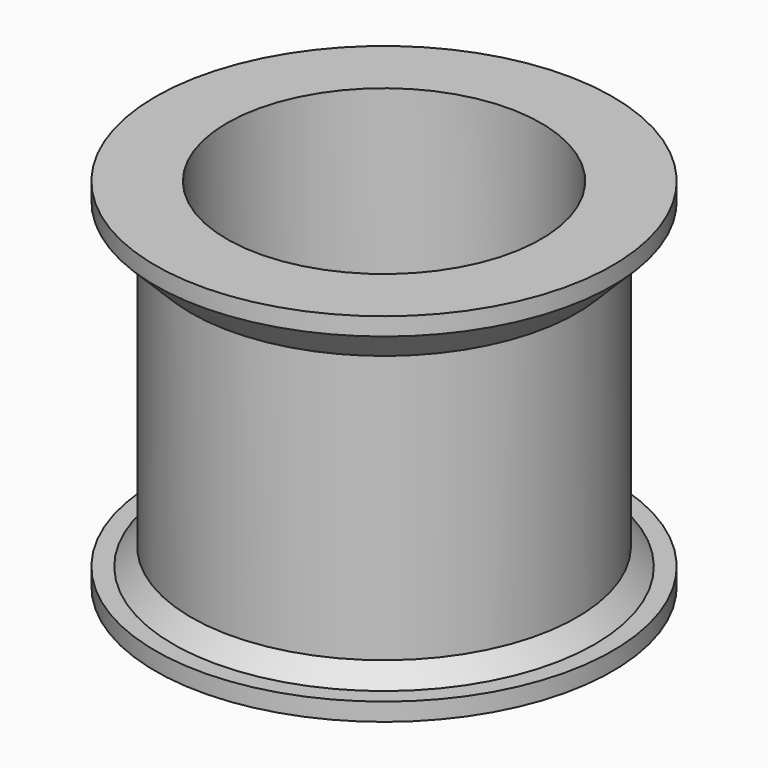
from build123d import *

# Parameters (mm, degrees)
F0_R     = 15.875
F0_R_2   = 4.318
F1_DEPTH = 11.43
F5_SIZE  = 1.5875
F4_R     = 15.875
F4_R_2   = 13.97
F6_DEPTH = 3.175


with BuildPart() as f1:
    # F0 (on Top) → F1 (new body)
    with BuildSketch(Plane.XY):
        Circle(F0_R)
        Circle(F0_R_2, mode=Mode.SUBTRACT)
    extrude(amount=F1_DEPTH)

    # F2 (on Front) → F3 (revolve)
    with BuildSketch(Plane.XZ):
        Polygon((-20.32, 0), (-10.16, 0), (-10.16, 1.5875), (-13.97, 1.5875), (-13.97, 31.75), (-20.32, 31.75), (-20.32, 30.1625), (-17.145, 30.1625), (-17.145, 26.9875), (-17.145, 1.5875), (-20.32, 1.5875), align=None)
        Polygon((-20.32, 30.1625), (-17.145, 26.9875), (-17.145, 30.1625), align=None)
    revolve(axis=Axis((0, 0, 11.5776285529), (0, 0, 1)))

    # F5
    f5_edges = [f1.edges().sort_by_distance(p)[0] for p in [
        (17.145, 0, 1.5875),
    ]]
    chamfer(f5_edges, length=F5_SIZE)

    # F4 (on face) → F6 (join)
    with BuildSketch(Plane.XY.offset(11.43)):
        Circle(F4_R)
        Circle(F4_R_2, mode=Mode.SUBTRACT)
        Circle(F4_R_2)
        with BuildLine():
            ThreePointArc((0, 13.49375), (1.9203608066, 13.3564030875), (3.8016286067, 12.9471583368))
            ThreePointArc((3.8016286067, 12.9471583368), (7.2952719665, 11.3516648998), (10.1978957754, 8.836527079))
            ThreePointArc((10.1978957754, 8.836527079), (12.2743466965, 5.6055064211), (13.3564030629, 1.9203609777))
            ThreePointArc((13.3564030629, 1.9203609777), (13.4593694669, 0.9626331682), (13.49375, 0))
            ThreePointArc((13.49375, 0), (13.1853755264, -2.8683028589), (12.2743467518, -5.6055063))
            ThreePointArc((12.2743467518, -5.6055063), (10.197895881, -8.836526957), (7.2952721608, -11.3516647749))
            ThreePointArc((7.2952721608, -11.3516647749), (3.8016288023, -12.9471582794), (8.16e-08, -13.49375))
            ThreePointArc((8.16e-08, -13.49375), (-3.8016286419, -12.9471583265), (-7.2952720168, -11.3516648675))
            ThreePointArc((-7.2952720168, -11.3516648675), (-10.1978957807, -8.8365270728), (-12.2743466957, -5.6055064229))
            ThreePointArc((-12.2743466957, -5.6055064229), (-13.3564030713, -1.920360919), (-13.3564030873, 1.9203608081))
            ThreePointArc((-13.3564030873, 1.9203608081), (-12.2743467595, 5.6055062831), (-10.1978958619, 8.8365269791))
            ThreePointArc((-10.1978958619, 8.8365269791), (-7.2952721155, 11.3516648041), (-3.8016288198, 12.9471582743))
            ThreePointArc((-3.8016288198, 12.9471582743), (-1.9203609165, 13.3564030717), (0, 13.49375))
        make_face(mode=Mode.SUBTRACT)
        with BuildLine():
            ThreePointArc((10.1978957754, 8.836527079), (7.2952719665, 11.3516648998), (3.8016286067, 12.9471583368))
            ThreePointArc((3.8016286067, 12.9471583368), (4.0909657389, 12.766807831), (4.2453187505, 12.462805481))
            Line((4.2453187505, 12.462805481), (4.8828478786, 9.2855481142))
            ThreePointArc((4.8828478786, 9.2855481142), (6.002488465, 10.799178406), (7.3980285057, 9.5353984813))
            ThreePointArc((7.3980285057, 9.5353984813), (7.1233157795, 8.7465364892), (6.4180233992, 8.2989507623))
            Line((6.4180233992, 8.2989507623), (9.572997339, 9.0389143838))
            ThreePointArc((9.572997339, 9.0389143838), (9.9136481809, 9.0247970952), (10.1978957754, 8.836527079))
        make_face()
        with BuildLine():
            ThreePointArc((13.3564030629, 1.9203609777), (12.2743466965, 5.6055064211), (10.1978957754, 8.836527079))
            ThreePointArc((10.1978957754, 8.836527079), (10.3129578638, 8.6426002713), (10.3529947858, 8.4206905243))
            ThreePointArc((10.3529947858, 8.4206905243), (10.3419731231, 8.302893943), (10.3092907399, 8.1891865402))
            Line((10.3092907399, 8.1891865402), (9.1278593511, 5.1716332867))
            ThreePointArc((9.1278593511, 5.1716332867), (10.5460444219, 5.9565819932), (11.5804512593, 4.7086253186))
            ThreePointArc((11.5804512593, 4.7086253186), (11.0431742993, 3.6713129516), (9.8859363825, 3.5116762306))
            Line((9.8859363825, 3.5116762306), (12.9401238926, 2.4284655514))
            ThreePointArc((12.9401238926, 2.4284655514), (13.2190652142, 2.2324196075), (13.3564030629, 1.9203609777))
        make_face()
        with BuildLine():
            ThreePointArc((-4.2453189127, 12.4628054073), (-4.090965925, 12.7668077529), (-3.8016288198, 12.9471582743))
            ThreePointArc((-3.8016288198, 12.9471582743), (-7.2952721155, 11.3516648041), (-10.1978958619, 8.8365269791))
            ThreePointArc((-10.1978958619, 8.8365269791), (-9.9136482865, 9.0247969722), (-9.5729974735, 9.0389142669))
            Line((-9.5729974735, 9.0389142669), (-6.4180233441, 8.2989507494))
            ThreePointArc((-6.4180233441, 8.2989507494), (-6.9168905199, 10.5306857375), (-4.8580285057, 9.5353984813))
            ThreePointArc((-4.8580285057, 9.5353984813), (-4.8642485781, 9.4098584688), (-4.8828478674, 9.2855481697))
            Line((-4.8828478674, 9.2855481697), (-4.2453189127, 12.4628054073))
        make_face()
        with BuildLine():
            ThreePointArc((13.49375, 0), (13.4593694669, 0.9626331682), (13.3564030629, 1.9203609777))
            ThreePointArc((13.3564030629, 1.9203609777), (13.3612485452, 1.8752914129), (13.3628664542, 1.8299910074))
            ThreePointArc((13.3628664542, 1.8299910074), (13.2933821525, 1.541171003), (13.1001357613, 1.315558735))
            Line((13.1001357613, 1.315558735), (10.474839974, -0.5842385682))
            ThreePointArc((10.474839974, -0.5842385682), (11.7970185973, -0.4820717165), (12.4893785884, -1.6131031131))
            ThreePointArc((12.4893785884, -1.6131031131), (11.6301765314, -2.8148289762), (10.2151344151, -2.390530692))
            Line((10.2151344151, -2.390530692), (12.1988525408, -4.9530039347))
            ThreePointArc((12.1988525408, -4.9530039347), (12.2975933857, -5.1363187527), (12.3317304542, -5.3417177242))
            ThreePointArc((12.3317304542, -5.3417177242), (12.3172187091, -5.4766967059), (12.2743467518, -5.6055063))
            ThreePointArc((12.2743467518, -5.6055063), (13.1853755264, -2.8683028589), (13.49375, 0))
        make_face()
        with BuildLine():
            ThreePointArc((-10.3092908365, 8.1891863905), (-10.3437969109, 8.5283789982), (-10.1978958619, 8.8365269791))
            ThreePointArc((-10.1978958619, 8.8365269791), (-12.2743467595, 5.6055062831), (-13.3564030873, 1.9203608081))
            ThreePointArc((-13.3564030873, 1.9203608081), (-13.219065249, 2.2324194318), (-12.9401239425, 2.4284653804))
            Line((-12.9401239425, 2.4284653804), (-9.8859363292, 3.5116762495))
            ThreePointArc((-9.8859363292, 3.5116762495), (-11.4656839052, 5.2362023594), (-9.1278593717, 5.1716333395))
            Line((-9.1278593717, 5.1716333395), (-10.3092908365, 8.1891863905))
        make_face()
        with BuildLine():
            ThreePointArc((-13.1001357616, 1.3155585568), (-13.3125454921, 1.5822501552), (-13.3564030873, 1.9203608081))
            ThreePointArc((-13.3564030873, 1.9203608081), (-13.3564030713, -1.920360919), (-12.2743466957, -5.6055064229))
            ThreePointArc((-12.2743466957, -5.6055064229), (-12.3275224114, -5.2687355378), (-12.1988524903, -4.9530041056))
            Line((-12.1988524903, -4.9530041056), (-10.2151343804, -2.3905306473))
            ThreePointArc((-10.2151343804, -2.3905306473), (-12.4764518155, -1.7938429858), (-10.4748400199, -0.584238535))
            Line((-10.4748400199, -0.584238535), (-13.1001357616, 1.3155585568))
        make_face()
        with BuildLine():
            ThreePointArc((7.2952721608, -11.3516647749), (10.197895881, -8.836526957), (12.2743467518, -5.6055063))
            ThreePointArc((12.2743467518, -5.6055063), (12.054654987, -5.8662318125), (11.7317802397, -5.9757496733))
            Line((11.7317802397, -5.9757496733), (8.4961329169, -6.1546188058))
            ThreePointArc((8.4961329169, -6.1546188058), (9.439122385, -6.5002060227), (9.8362324879, -7.4226827041))
            ThreePointArc((9.8362324879, -7.4226827041), (8.6218249278, -8.6914653808), (7.3010994475, -7.5337610106))
            Line((7.3010994475, -7.5337610106), (7.5845317003, -10.7619296679))
            ThreePointArc((7.5845317003, -10.7619296679), (7.5863565184, -10.7896726012), (7.5869651801, -10.8174688212))
            ThreePointArc((7.5869651801, -10.8174688212), (7.509291356, -11.1217918956), (7.2952721608, -11.3516647749))
        make_face()
        with BuildLine():
            ThreePointArc((-11.7317801436, -5.9757498234), (-12.0546549192, -5.866231961), (-12.2743466957, -5.6055064229))
            ThreePointArc((-12.2743466957, -5.6055064229), (-10.1978957807, -8.8365270728), (-7.2952720168, -11.3516648675))
            ThreePointArc((-7.2952720168, -11.3516648675), (-7.52207831, -11.0971041407), (-7.5845315655, -10.7619297844))
            Line((-7.5845315655, -10.7619297844), (-7.3010994426, -7.5337609542))
            ThreePointArc((-7.3010994426, -7.5337609542), (-9.5260344288, -8.2543558576), (-8.4961329734, -6.1546188027))
            Line((-8.4961329734, -6.1546188027), (-11.7317801436, -5.9757498234))
        make_face()
        with BuildLine():
            ThreePointArc((8.16e-08, -13.49375), (3.8016288023, -12.9471582794), (7.2952721608, -11.3516647749))
            ThreePointArc((7.2952721608, -11.3516647749), (6.9694967924, -11.4522267613), (6.6386673847, -11.369799783))
            Line((6.6386673847, -11.369799783), (3.8199636894, -9.770951059))
            ThreePointArc((3.8199636894, -9.770951059), (4.2907915357, -10.2364245911), (4.4633680987, -10.8756129827))
            ThreePointArc((4.4633680987, -10.8756129827), (2.8892512665, -12.1086632462), (2.0690169925, -10.2850754393))
            Line((2.0690169925, -10.2850754393), (0.5621756347, -13.1540187717))
            ThreePointArc((0.5621756347, -13.1540187717), (0.3284276459, -13.4022206386), (8.16e-08, -13.49375))
        make_face()
        with BuildLine():
            ThreePointArc((-6.6386672228, -11.3697998573), (-6.969496637, -11.4522268501), (-7.2952720168, -11.3516648675))
            ThreePointArc((-7.2952720168, -11.3516648675), (-3.8016286419, -12.9471583265), (8.16e-08, -13.49375))
            ThreePointArc((8.16e-08, -13.49375), (-0.3284274706, -13.4022206459), (-0.5621754583, -13.1540187967))
            Line((-0.5621754583, -13.1540187967), (-2.0690170188, -10.2850753892))
            ThreePointArc((-2.0690170188, -10.2850753892), (-1.9603178419, -10.571496123), (-1.9233680987, -10.8756129827))
            ThreePointArc((-1.9233680987, -10.8756129827), (-3.8325564657, -11.973036434), (-3.8199637387, -9.7709510869))
            Line((-3.8199637387, -9.7709510869), (-6.6386672228, -11.3697998573))
        make_face()
        with BuildLine():
            ThreePointArc((7.3980285057, 9.5353984813), (6.002488465, 10.799178406), (4.8828478786, 9.2855481142))
            ThreePointArc((4.8828478786, 9.2855481142), (5.4414146913, 8.4670064793), (6.4180233992, 8.2989507623))
            ThreePointArc((6.4180233992, 8.2989507623), (7.1233157795, 8.7465364892), (7.3980285057, 9.5353984813))
        make_face()
        with BuildLine():
            ThreePointArc((-6.4180233441, 8.2989507494), (-5.4414146437, 8.4670065099), (-4.8828478674, 9.2855481697))
            ThreePointArc((-4.8828478674, 9.2855481697), (-4.8642485781, 9.4098584688), (-4.8580285057, 9.5353984813))
            ThreePointArc((-4.8580285057, 9.5353984813), (-6.9168905199, 10.5306857375), (-6.4180233441, 8.2989507494))
        make_face()
        with BuildLine():
            ThreePointArc((9.1278593511, 5.1716332867), (9.155218637, 4.1810482264), (9.8859363825, 3.5116762306))
            ThreePointArc((9.8859363825, 3.5116762306), (11.0431742993, 3.6713129516), (11.5804512593, 4.7086253186))
            ThreePointArc((11.5804512593, 4.7086253186), (10.5460444219, 5.9565819932), (9.1278593511, 5.1716332867))
        make_face()
        with BuildLine():
            ThreePointArc((-9.0404512593, 4.7086253186), (-9.06249459, 4.944218509), (-9.1278593717, 5.1716333395))
            ThreePointArc((-9.1278593717, 5.1716333395), (-11.4656839052, 5.2362023594), (-9.8859363292, 3.5116762495))
            ThreePointArc((-9.8859363292, 3.5116762495), (-9.273138876, 3.9759023018), (-9.0404512593, 4.7086253186))
        make_face()
        with BuildLine():
            ThreePointArc((12.4893785884, -1.6131031131), (11.7970185973, -0.4820717165), (10.474839974, -0.5842385682))
            ThreePointArc((10.474839974, -0.5842385682), (9.9623053531, -1.4323632965), (10.2151344151, -2.390530692))
            ThreePointArc((10.2151344151, -2.390530692), (11.6301765314, -2.8148289762), (12.4893785884, -1.6131031131))
        make_face()
        with BuildLine():
            ThreePointArc((-9.9493785884, -1.6131031131), (-10.0883472046, -1.035463079), (-10.4748400199, -0.584238535))
            ThreePointArc((-10.4748400199, -0.584238535), (-12.4764518155, -1.7938429858), (-10.2151343804, -2.3905306473))
            ThreePointArc((-10.2151343804, -2.3905306473), (-10.0176527161, -2.0239010293), (-9.9493785884, -1.6131031131))
        make_face()
        with BuildLine():
            ThreePointArc((9.8362324879, -7.4226827041), (9.439122385, -6.5002060227), (8.4961329169, -6.1546188058))
            ThreePointArc((8.4961329169, -6.1546188058), (7.6064305099, -6.5910095934), (7.3010994475, -7.5337610106))
            ThreePointArc((7.3010994475, -7.5337610106), (8.6218249278, -8.6914653808), (9.8362324879, -7.4226827041))
        make_face()
        with BuildLine():
            ThreePointArc((-7.2962324879, -7.4226827041), (-7.643755826, -6.5497927865), (-8.4961329734, -6.1546188027))
            ThreePointArc((-8.4961329734, -6.1546188027), (-9.5260344288, -8.2543558576), (-7.3010994426, -7.5337609542))
            ThreePointArc((-7.3010994426, -7.5337609542), (-7.29744981, -7.4782751157), (-7.2962324879, -7.4226827041))
        make_face()
        with BuildLine():
            ThreePointArc((4.4633680987, -10.8756129827), (4.2907915357, -10.2364245911), (3.8199636894, -9.770951059))
            ThreePointArc((3.8199636894, -9.770951059), (2.8355677243, -9.6570569142), (2.0690169925, -10.2850754393))
            ThreePointArc((2.0690169925, -10.2850754393), (2.8892512665, -12.1086632462), (4.4633680987, -10.8756129827))
        make_face()
        with BuildLine():
            ThreePointArc((-2.0690170188, -10.2850753892), (-2.8355677786, -9.6570568982), (-3.8199637387, -9.7709510869))
            ThreePointArc((-3.8199637387, -9.7709510869), (-3.8325564657, -11.973036434), (-1.9233680987, -10.8756129827))
            ThreePointArc((-1.9233680987, -10.8756129827), (-1.9603178419, -10.571496123), (-2.0690170188, -10.2850753892))
        make_face()
        with BuildLine():
            ThreePointArc((3.1665117699, 12.7795717652), (3.4607178673, 12.9518652935), (3.8016286067, 12.9471583368))
            ThreePointArc((3.8016286067, 12.9471583368), (1.9203608066, 13.3564030875), (0, 13.49375))
            Line((0, 13.49375), (0, 12.60475))
            ThreePointArc((0, 12.60475), (0.8980256121, 12.2327756121), (1.27, 11.33475))
            ThreePointArc((1.27, 11.33475), (1.177219252, 10.8582472899), (0.9124333342, 10.4513670646))
            Line((0.9124333342, 10.4513670646), (3.1665117699, 12.7795717652))
        make_face()
        with BuildLine():
            Line((0, 12.60475), (0, 13.49375))
            ThreePointArc((0, 13.49375), (-1.9203609165, 13.3564030717), (-3.8016288198, 12.9471582743))
            ThreePointArc((-3.8016288198, 12.9471582743), (-3.4607180661, 12.9518652586), (-3.1665119462, 12.7795717395))
            Line((-3.1665119462, 12.7795717395), (-0.9124332948, 10.4513670239))
            ThreePointArc((-0.9124332948, 10.4513670239), (-1.1693580247, 11.8302313924), (0, 12.60475))
        make_face()
        with BuildLine():
            ThreePointArc((1.27, 11.33475), (0.8980256121, 12.2327756121), (0, 12.60475))
            Line((0, 12.60475), (0, 10.06475))
            ThreePointArc((0, 10.06475), (0.4954814184, 10.1653919864), (0.9124333342, 10.4513670646))
            ThreePointArc((0.9124333342, 10.4513670646), (1.177219252, 10.8582472899), (1.27, 11.33475))
        make_face()
        with BuildLine():
            Line((0, 10.06475), (0, 12.60475))
            ThreePointArc((0, 12.60475), (-1.1693580247, 11.8302313924), (-0.9124332948, 10.4513670239))
            ThreePointArc((-0.9124332948, 10.4513670239), (-0.4954813924, 10.1653919753), (0, 10.06475))
        make_face()
    extrude(amount=F6_DEPTH)


solid = f1.part
